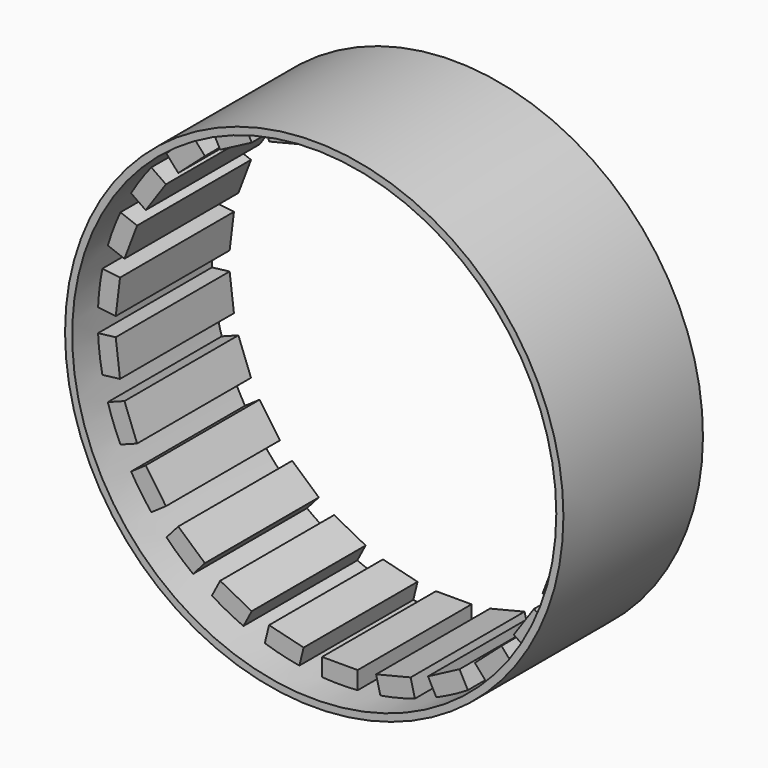
from build123d import *

# Parameters (mm, degrees)
F0_R     = 70
F1_DEPTH = 40
F2_COUNT = 26
F4_R     = 70
F4_R_2   = 68
F5_DEPTH = 9


with BuildPart() as f1:
    # F0 (on Front) → F1 (new body)
    with BuildSketch(Plane.XZ):
        Circle(F0_R)
        with BuildLine():
            ThreePointArc((5, 67.8159273327), (49.8196748283, 46.2817458616), (68, 0))
            ThreePointArc((68, 0), (-46.2817458616, -49.8196748283), (-5, 67.8159273327))
            ThreePointArc((-5, 67.8159273327), (0, 68), (5, 67.8159273327))
        make_face(mode=Mode.SUBTRACT)
        with BuildLine():
            Line((5, 62.8159273327), (5, 67.8159273327))
            ThreePointArc((5, 67.8159273327), (0, 68), (-5, 67.8159273327))
            Line((-5, 67.8159273327), (-5, 62.8159273327))
            Line((-5, 62.8159273327), (5, 62.8159273327))
        make_face()
    extrude(amount=F1_DEPTH)


with BuildPart() as f2_1:
    # F2: instance of F1
    add(f1.part.rotate(Axis((0, 0, 0), (0, 1, 0)), 1 * 360 / F2_COUNT))


with BuildPart() as f2_2:
    # F2: instance of F1
    add(f1.part.rotate(Axis((0, 0, 0), (0, 1, 0)), 2 * 360 / F2_COUNT))


with BuildPart() as f2_3:
    # F2: instance of F1
    add(f1.part.rotate(Axis((0, 0, 0), (0, 1, 0)), 3 * 360 / F2_COUNT))


with BuildPart() as f2_4:
    # F2: instance of F1
    add(f1.part.rotate(Axis((0, 0, 0), (0, 1, 0)), 4 * 360 / F2_COUNT))


with BuildPart() as f2_5:
    # F2: instance of F1
    add(f1.part.rotate(Axis((0, 0, 0), (0, 1, 0)), 5 * 360 / F2_COUNT))


with BuildPart() as f2_6:
    # F2: instance of F1
    add(f1.part.rotate(Axis((0, 0, 0), (0, 1, 0)), 6 * 360 / F2_COUNT))


with BuildPart() as f2_7:
    # F2: instance of F1
    add(f1.part.rotate(Axis((0, 0, 0), (0, 1, 0)), 7 * 360 / F2_COUNT))


with BuildPart() as f2_8:
    # F2: instance of F1
    add(f1.part.rotate(Axis((0, 0, 0), (0, 1, 0)), 8 * 360 / F2_COUNT))


with BuildPart() as f2_9:
    # F2: instance of F1
    add(f1.part.rotate(Axis((0, 0, 0), (0, 1, 0)), 9 * 360 / F2_COUNT))


with BuildPart() as f2_10:
    # F2: instance of F1
    add(f1.part.rotate(Axis((0, 0, 0), (0, 1, 0)), 10 * 360 / F2_COUNT))


with BuildPart() as f2_11:
    # F2: instance of F1
    add(f1.part.rotate(Axis((0, 0, 0), (0, 1, 0)), 11 * 360 / F2_COUNT))


with BuildPart() as f2_12:
    # F2: instance of F1
    add(f1.part.rotate(Axis((0, 0, 0), (0, 1, 0)), 12 * 360 / F2_COUNT))


with BuildPart() as f2_13:
    # F2: instance of F1
    add(f1.part.rotate(Axis((0, 0, 0), (0, 1, 0)), 13 * 360 / F2_COUNT))


with BuildPart() as f2_14:
    # F2: instance of F1
    add(f1.part.rotate(Axis((0, 0, 0), (0, 1, 0)), 14 * 360 / F2_COUNT))


with BuildPart() as f2_15:
    # F2: instance of F1
    add(f1.part.rotate(Axis((0, 0, 0), (0, 1, 0)), 15 * 360 / F2_COUNT))


with BuildPart() as f2_16:
    # F2: instance of F1
    add(f1.part.rotate(Axis((0, 0, 0), (0, 1, 0)), 16 * 360 / F2_COUNT))


with BuildPart() as f2_17:
    # F2: instance of F1
    add(f1.part.rotate(Axis((0, 0, 0), (0, 1, 0)), 17 * 360 / F2_COUNT))


with BuildPart() as f2_18:
    # F2: instance of F1
    add(f1.part.rotate(Axis((0, 0, 0), (0, 1, 0)), 18 * 360 / F2_COUNT))


with BuildPart() as f2_19:
    # F2: instance of F1
    add(f1.part.rotate(Axis((0, 0, 0), (0, 1, 0)), 19 * 360 / F2_COUNT))


with BuildPart() as f2_20:
    # F2: instance of F1
    add(f1.part.rotate(Axis((0, 0, 0), (0, 1, 0)), 20 * 360 / F2_COUNT))


with BuildPart() as f2_21:
    # F2: instance of F1
    add(f1.part.rotate(Axis((0, 0, 0), (0, 1, 0)), 21 * 360 / F2_COUNT))


with BuildPart() as f2_22:
    # F2: instance of F1
    add(f1.part.rotate(Axis((0, 0, 0), (0, 1, 0)), 22 * 360 / F2_COUNT))


with BuildPart() as f2_23:
    # F2: instance of F1
    add(f1.part.rotate(Axis((0, 0, 0), (0, 1, 0)), 23 * 360 / F2_COUNT))


with BuildPart() as f2_24:
    # F2: instance of F1
    add(f1.part.rotate(Axis((0, 0, 0), (0, 1, 0)), 24 * 360 / F2_COUNT))


with BuildPart() as f2_25:
    # F2: instance of F1
    add(f1.part.rotate(Axis((0, 0, 0), (0, 1, 0)), 25 * 360 / F2_COUNT))


with BuildPart() as f2_3_1:
    add(f2_3.part)

    # F3: union F2_4, F2_6, F2_10, F2_8, F2_11, F2_12, F2_9, F2_2, F2_15, F2_13, F2_16, F2_14, F2_19, F2_18, F2_17, F2_7, F2_23, F2_22, F2_21, F2_20, F2_24, F2_1, F1, F2_25, F2_5
    add(f2_4.part)
    add(f2_6.part)
    add(f2_10.part)
    add(f2_8.part)
    add(f2_11.part)
    add(f2_12.part)
    add(f2_9.part)
    add(f2_2.part)
    add(f2_15.part)
    add(f2_13.part)
    add(f2_16.part)
    add(f2_14.part)
    add(f2_19.part)
    add(f2_18.part)
    add(f2_17.part)
    add(f2_7.part)
    add(f2_23.part)
    add(f2_22.part)
    add(f2_21.part)
    add(f2_20.part)
    add(f2_24.part)
    add(f2_1.part)
    add(f1.part)
    add(f2_25.part)
    add(f2_5.part)

    # F4 (on face) → F5 (join)
    with BuildSketch(Plane.XZ.offset(40)):
        Circle(F4_R)
        Circle(F4_R_2, mode=Mode.SUBTRACT)
    extrude(amount=F5_DEPTH)


solid = f2_3_1.part
